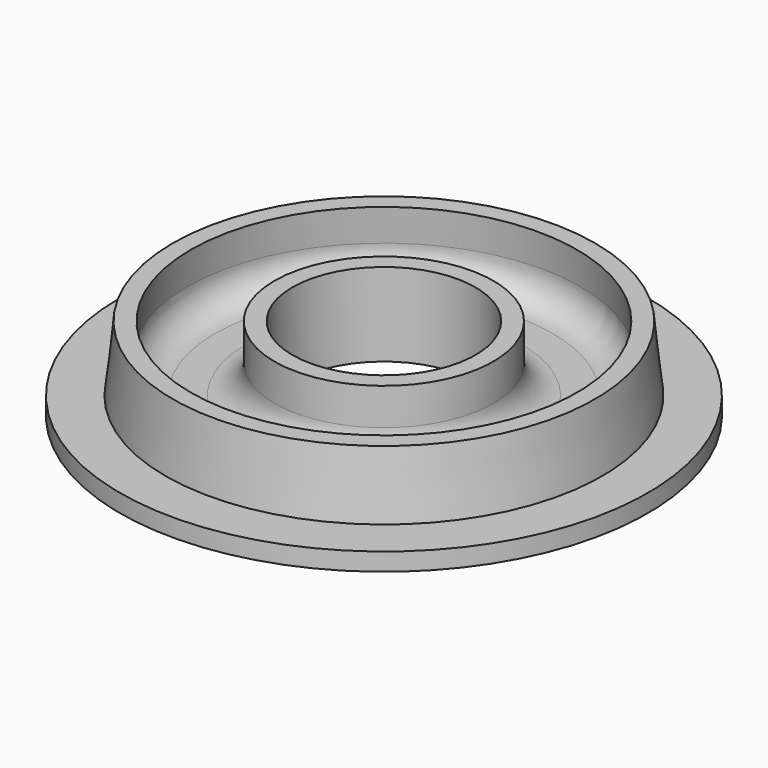
from build123d import *

# Parameters (mm, degrees)
F2_T = -3.175
F3_R = 5.08
F4_R = 5.08


with BuildPart() as f1:
    # F0 (on Front) → F1 (revolve)
    with BuildSketch(Plane.XZ):
        Polygon((-16.3068, 2.9675877146), (-16.3068, 17.7895731165), (-37.592, 17.7895731165), (-38.862, 6.1425877146), (-46.99, 6.1425877146), (-46.99, 2.9675877146), align=None)
    revolve(axis=Axis((0, 0, 15.8357990333), (0, 0, 1)))

    # F2
    f2_openings = [f1.faces().sort_by_distance(p)[0] for p in [
        (17.370062, 0, 17.789573),
    ]]
    offset(amount=F2_T, openings=f2_openings)

    # F3
    f3_edges = [f1.edges().sort_by_distance(p)[0] for p in [
        (19.4818, 0, 6.142588),
    ]]
    fillet(f3_edges, radius=F3_R)

    # F4
    f4_edges = [f1.edges().sort_by_distance(p)[0] for p in [
        (35.66818, 0, 6.142588),
    ]]
    fillet(f4_edges, radius=F4_R)


solid = f1.part
